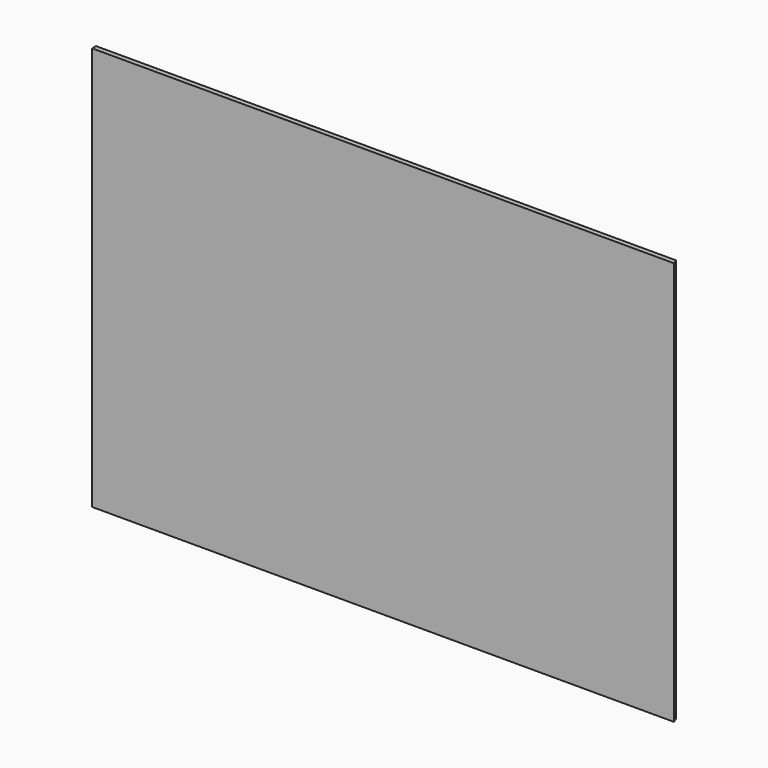
from build123d import *

# Parameters (mm, degrees)
F0_W     = 1519.0471722421
F0_H     = 1054.1
F1_DEPTH = 12.7
F2_SIZE2 = 5.260502
F2_SIZE  = 12.69999


# Not quite as in the source:
# - a fillet or chamfer is up to 0.001 mm smaller than in the source, because OpenCascade refuses the exact size


with BuildPart() as f1:
    # F0 (on Front) → F1 (new body)
    with BuildSketch(Plane.XZ):
        with Locations((759.5235861211, 527.05)):
            Rectangle(F0_W, F0_H)
    extrude(amount=-F1_DEPTH)

    # F2 (size 12.7 and 5.2605122421 in the source; OpenCascade refuses exactly that, so slightly less here)
    f2_edges = [f1.edges().sort_by_distance(p)[0] for p in [
        (1519.047172, 12.7, 527.05),
    ]]
    f2_side = f1.faces().sort_by_distance((1519.047172, 6.35, 527.05))[0]
    chamfer(f2_edges, length=F2_SIZE, length2=F2_SIZE2, reference=f2_side)


solid = f1.part
